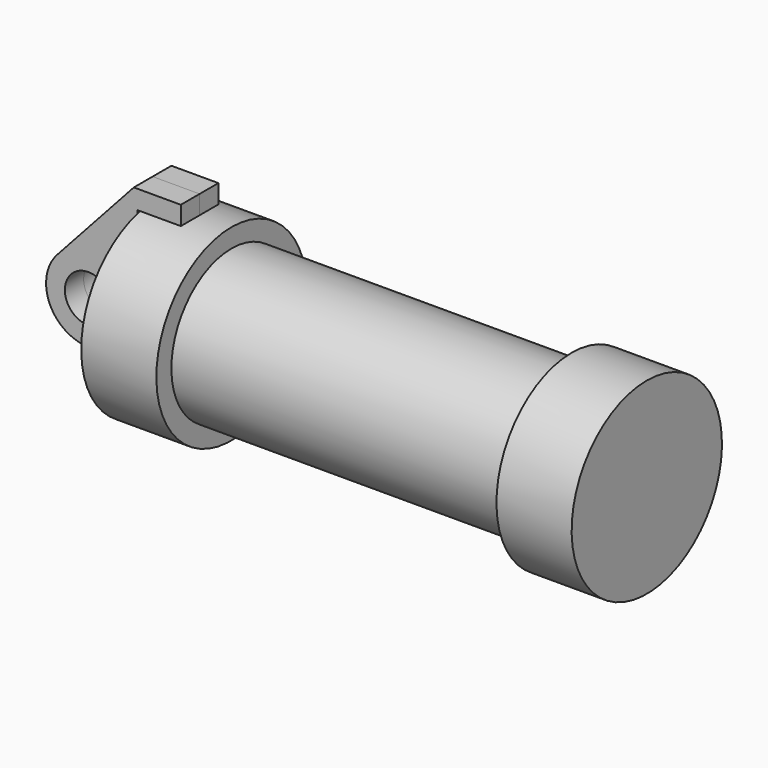
from build123d import *

# Parameters (mm, degrees)
F0_W     = 5.842
F0_H     = 12.7
F0_R     = 3.175
F3_DEPTH = 3.175


# Not quite as in the source:
# - a feature of the source that left no trace in its solid (it failed there, or was rolled back) is left out


with BuildPart() as f1:
    # F0 (on Front) → F1 (revolve)
    with BuildSketch(Plane.XZ):
        Polygon((5.842, 12.7), (5.842, 0), (66.294, 0), (66.294, 12.7), (56.134, 12.7), (56.134, 10.16), (10.16, 10.16), (10.16, 12.7), align=None)
        with Locations((2.921, 6.35)):
            Rectangle(F0_W, F0_H)
    revolve(axis=Axis((33.147, 0, 0), (-1, 0, 0)))


with BuildPart() as f3:
    # F0 (on Front) → F3 (new body, symmetric)
    with BuildSketch(Plane.XZ):
        with BuildLine():
            ThreePointArc((-8.1826630726, -5.5069827884), (-3.1957909266, -4.5493385486), (-0.9398, 0))
            ThreePointArc((-0.9398, 0), (-4.5919612295, 5.3297205562), (-10.8806298187, 3.8475430269))
            ThreePointArc((-10.8806298187, 3.8475430269), (-12.1459778134, -1.5837270034), (-8.1826630726, -5.5069827884))
        make_face()
        with Locations((-6.6548, 0)):
            Circle(F0_R, mode=Mode.SUBTRACT)
        with BuildLine():
            Line((-0.9398, 0), (0, 0))
            Line((0, 0), (0, 12.7))
            Line((0, 12.7), (5.842, 12.7))
            Line((5.842, 12.7), (5.842, 15.24))
            Line((5.842, 15.24), (-0.508, 15.24))
            Line((-0.508, 15.24), (-10.8806298187, 3.8475430269))
            ThreePointArc((-10.8806298187, 3.8475430269), (-4.5919612295, 5.3297205562), (-0.9398, 0))
        make_face()
    extrude(amount=F3_DEPTH, both=True)


with BuildPart() as f3b:
    # F2 (on face) → F3, piece 2 (new body, symmetric)
    with BuildSketch(Plane.XZ):
        with BuildLine():
            Line((5.842, -9.398), (5.842, 0))
            Line((5.842, 0), (0, 0))
            Line((0, 0), (-0.9398, 0))
            ThreePointArc((-0.9398, 0), (-3.1957909266, -4.5493385486), (-8.1826630726, -5.5069827884))
            Line((-8.1826630726, -5.5069827884), (5.842, -9.398))
        make_face()
    extrude(amount=F3_DEPTH, both=True)


solid = Compound([f1.part, f3.part, f3b.part])
